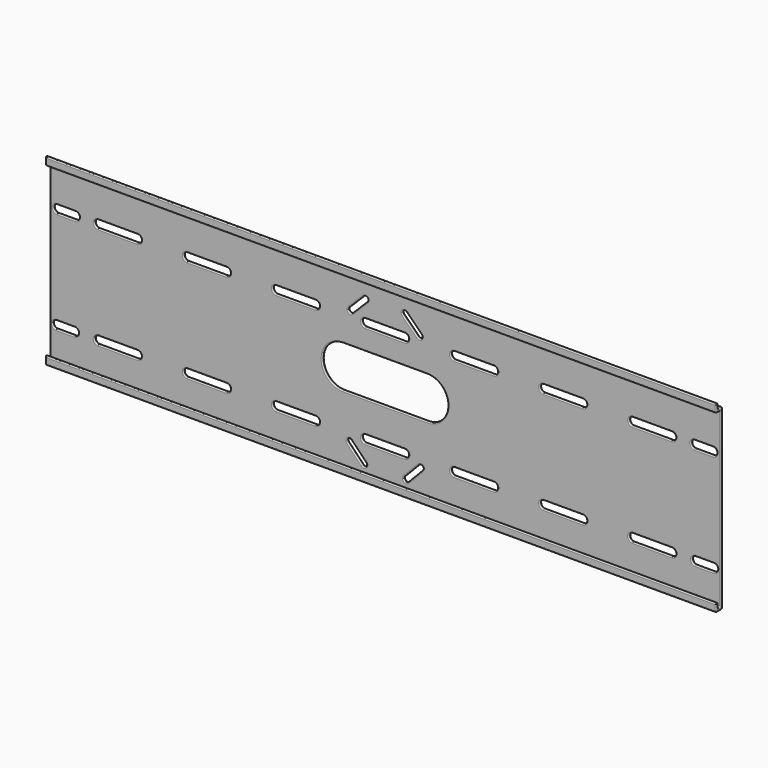
from build123d import *

# Parameters (mm, degrees)
F0_W     = 812.8
F0_H     = 222.25
F1_DEPTH = 9.525
F2_W     = 3.175
F2_H     = 6.35
F2_W_2   = 6.35
F3_DEPTH = 812.801
F5_DEPTH = 9.526
F6_F1_R  = 1.27
F6_F2_R  = 1.27


with BuildPart() as f1:
    # F0 (on Front) → F1 (new body)
    with BuildSketch(Plane.XZ):
        with Locations((103.5543584931, 7.2905048728)):
            Rectangle(F0_W, F0_H)
        with BuildLine():
            ThreePointArc((-294.9081415069, -65.7344951272), (-299.6706415069, -60.9719951272), (-294.9081415069, -56.2094951272))
            Line((-294.9081415069, -56.2094951272), (-272.6831415069, -56.2094951272))
            ThreePointArc((-272.6831415069, -56.2094951272), (-269.3155454615, -57.6043990818), (-267.9206415069, -60.9719951272))
            ThreePointArc((-267.9206415069, -60.9719951272), (-269.3155454615, -64.3395911726), (-272.6831415069, -65.7344951272))
            Line((-272.6831415069, -65.7344951272), (-294.9081415069, -65.7344951272))
        make_face(mode=Mode.SUBTRACT)
        with BuildLine():
            ThreePointArc((-191.7550515069, -60.9719951272), (-193.1499554615, -64.3395911726), (-196.5175515069, -65.7344951272))
            Line((-196.5175515069, -65.7344951272), (-244.1425515069, -65.7344951272))
            ThreePointArc((-244.1425515069, -65.7344951272), (-248.9050515069, -60.9719951272), (-244.1425515069, -56.2094951272))
            Line((-244.1425515069, -56.2094951272), (-196.5175515069, -56.2094951272))
            ThreePointArc((-196.5175515069, -56.2094951272), (-193.1499554615, -57.6043990818), (-191.7550515069, -60.9719951272))
        make_face(mode=Mode.SUBTRACT)
        with BuildLine():
            ThreePointArc((-83.7935815069, -60.9719951272), (-85.1884854615, -64.3395911726), (-88.5560815069, -65.7344951272))
            Line((-88.5560815069, -65.7344951272), (-136.1810815069, -65.7344951272))
            ThreePointArc((-136.1810815069, -65.7344951272), (-140.9435815069, -60.9719951272), (-136.1810815069, -56.2094951272))
            Line((-136.1810815069, -56.2094951272), (-88.5560815069, -56.2094951272))
            ThreePointArc((-88.5560815069, -56.2094951272), (-85.1884854615, -57.6043990818), (-83.7935815069, -60.9719951272))
        make_face(mode=Mode.SUBTRACT)
        with BuildLine():
            ThreePointArc((24.1678884931, -60.9719951272), (22.7729845385, -64.3395911726), (19.4053884931, -65.7344951272))
            Line((19.4053884931, -65.7344951272), (-28.2196115069, -65.7344951272))
            ThreePointArc((-28.2196115069, -65.7344951272), (-32.9821115069, -60.9719951272), (-28.2196115069, -56.2094951272))
            Line((-28.2196115069, -56.2094951272), (19.4053884931, -56.2094951272))
            ThreePointArc((19.4053884931, -56.2094951272), (22.7729845385, -57.6043990818), (24.1678884931, -60.9719951272))
        make_face(mode=Mode.SUBTRACT)
        with BuildLine():
            ThreePointArc((79.7418584931, -65.7344951272), (74.9793584931, -60.9719951272), (79.7418584931, -56.2094951272))
            Line((79.7418584931, -56.2094951272), (127.3668584931, -56.2094951272))
            ThreePointArc((127.3668584931, -56.2094951272), (130.7344545385, -57.6043990818), (132.1293584931, -60.9719951272))
            ThreePointArc((132.1293584931, -60.9719951272), (130.7344545385, -64.3395911726), (127.3668584931, -65.7344951272))
            Line((127.3668584931, -65.7344951272), (79.7418584931, -65.7344951272))
        make_face(mode=Mode.SUBTRACT)
        with BuildLine():
            Line((187.7033284931, -56.2094951272), (235.3283284931, -56.2094951272))
            ThreePointArc((235.3283284931, -56.2094951272), (238.6959245385, -57.6043990818), (240.0908284931, -60.9719951272))
            ThreePointArc((240.0908284931, -60.9719951272), (238.6959245385, -64.3395911726), (235.3283284931, -65.7344951272))
            Line((235.3283284931, -65.7344951272), (187.7033284931, -65.7344951272))
            ThreePointArc((187.7033284931, -65.7344951272), (182.9408284931, -60.9719951272), (187.7033284931, -56.2094951272))
        make_face(mode=Mode.SUBTRACT)
        with BuildLine():
            ThreePointArc((343.2897984931, -56.2094951272), (346.6573945385, -57.6043990818), (348.0522984931, -60.9719951272))
            ThreePointArc((348.0522984931, -60.9719951272), (346.6573945385, -64.3395911726), (343.2897984931, -65.7344951272))
            Line((343.2897984931, -65.7344951272), (295.6647984931, -65.7344951272))
            ThreePointArc((295.6647984931, -65.7344951272), (290.9022984931, -60.9719951272), (295.6647984931, -56.2094951272))
            Line((295.6647984931, -56.2094951272), (343.2897984931, -56.2094951272))
        make_face(mode=Mode.SUBTRACT)
        with BuildLine():
            ThreePointArc((451.2512684931, -56.2094951272), (454.6188645385, -57.6043990818), (456.0137684931, -60.9719951272))
            ThreePointArc((456.0137684931, -60.9719951272), (454.6188645385, -64.3395911726), (451.2512684931, -65.7344951272))
            Line((451.2512684931, -65.7344951272), (403.6262684931, -65.7344951272))
            ThreePointArc((403.6262684931, -65.7344951272), (398.8637684931, -60.9719951272), (403.6262684931, -56.2094951272))
            Line((403.6262684931, -56.2094951272), (451.2512684931, -56.2094951272))
        make_face(mode=Mode.SUBTRACT)
        with BuildLine():
            Line((479.7918584931, -56.2094951272), (502.0168584931, -56.2094951272))
            ThreePointArc((502.0168584931, -56.2094951272), (505.3844545385, -57.6043990818), (506.7793584931, -60.9719951272))
            ThreePointArc((506.7793584931, -60.9719951272), (505.3844545385, -64.3395911726), (502.0168584931, -65.7344951272))
            Line((502.0168584931, -65.7344951272), (479.7918584931, -65.7344951272))
            ThreePointArc((479.7918584931, -65.7344951272), (475.0293584931, -60.9719951272), (479.7918584931, -56.2094951272))
        make_face(mode=Mode.SUBTRACT)
        with BuildLine():
            ThreePointArc((-293.891865778, 58.0905048728), (-298.654365778, 62.8530048728), (-293.891865778, 67.6155048728))
            Line((-293.891865778, 67.6155048728), (-271.666865778, 67.6155048728))
            ThreePointArc((-271.666865778, 67.6155048728), (-268.2992697326, 66.2206009182), (-266.904365778, 62.8530048728))
            ThreePointArc((-266.904365778, 62.8530048728), (-268.2992697326, 59.4854088274), (-271.666865778, 58.0905048728))
            Line((-271.666865778, 58.0905048728), (-293.891865778, 58.0905048728))
        make_face(mode=Mode.SUBTRACT)
        with BuildLine():
            ThreePointArc((-196.4831415069, 67.6155048728), (-193.1155454615, 66.2206009182), (-191.7206415069, 62.8530048728))
            ThreePointArc((-191.7206415069, 62.8530048728), (-193.1155454615, 59.4854088274), (-196.4831415069, 58.0905048728))
            Line((-196.4831415069, 58.0905048728), (-244.1081415069, 58.0905048728))
            ThreePointArc((-244.1081415069, 58.0905048728), (-248.8706415069, 62.8530048728), (-244.1081415069, 67.6155048728))
            Line((-244.1081415069, 67.6155048728), (-196.4831415069, 67.6155048728))
        make_face(mode=Mode.SUBTRACT)
        with BuildLine():
            ThreePointArc((-88.5331415069, 67.6155048728), (-85.1655454615, 66.2206009182), (-83.7706415069, 62.8530048728))
            ThreePointArc((-83.7706415069, 62.8530048728), (-85.1655454615, 59.4854088274), (-88.5331415069, 58.0905048728))
            Line((-88.5331415069, 58.0905048728), (-136.1581415069, 58.0905048728))
            ThreePointArc((-136.1581415069, 58.0905048728), (-140.9206415069, 62.8530048728), (-136.1581415069, 67.6155048728))
            Line((-136.1581415069, 67.6155048728), (-88.5331415069, 67.6155048728))
        make_face(mode=Mode.SUBTRACT)
        with BuildLine():
            ThreePointArc((19.4168584931, 67.6155048728), (22.7844545385, 66.2206009182), (24.1793584931, 62.8530048728))
            ThreePointArc((24.1793584931, 62.8530048728), (22.7844545385, 59.4854088274), (19.4168584931, 58.0905048728))
            Line((19.4168584931, 58.0905048728), (-28.2081415069, 58.0905048728))
            ThreePointArc((-28.2081415069, 58.0905048728), (-32.9706415069, 62.8530048728), (-28.2081415069, 67.6155048728))
            Line((-28.2081415069, 67.6155048728), (19.4168584931, 67.6155048728))
        make_face(mode=Mode.SUBTRACT)
        with BuildLine():
            ThreePointArc((52.7543584931, -18.1094951272), (27.3543584931, 7.2905048728), (52.7543584931, 32.6905048728))
            Line((52.7543584931, 32.6905048728), (154.3543584931, 32.6905048728))
            ThreePointArc((154.3543584931, 32.6905048728), (172.3148707352, 25.2510171149), (179.7543584931, 7.2905048728))
            ThreePointArc((179.7543584931, 7.2905048728), (172.3148707352, -10.6700073693), (154.3543584931, -18.1094951272))
            Line((154.3543584931, -18.1094951272), (52.7543584931, -18.1094951272))
        make_face(mode=Mode.SUBTRACT)
        with BuildLine():
            ThreePointArc((79.7418584931, 58.0905048728), (74.9793584931, 62.8530048728), (79.7418584931, 67.6155048728))
            Line((79.7418584931, 67.6155048728), (127.3668584931, 67.6155048728))
            ThreePointArc((127.3668584931, 67.6155048728), (130.7344545385, 66.2206009182), (132.1293584931, 62.8530048728))
            ThreePointArc((132.1293584931, 62.8530048728), (130.7344545385, 59.4854088274), (127.3668584931, 58.0905048728))
            Line((127.3668584931, 58.0905048728), (79.7418584931, 58.0905048728))
        make_face(mode=Mode.SUBTRACT)
        with BuildLine():
            ThreePointArc((187.6918584931, 58.0905048728), (182.9293584931, 62.8530048728), (187.6918584931, 67.6155048728))
            Line((187.6918584931, 67.6155048728), (235.3168584931, 67.6155048728))
            ThreePointArc((235.3168584931, 67.6155048728), (238.6844545385, 66.2206009182), (240.0793584931, 62.8530048728))
            ThreePointArc((240.0793584931, 62.8530048728), (238.6844545385, 59.4854088274), (235.3168584931, 58.0905048728))
            Line((235.3168584931, 58.0905048728), (187.6918584931, 58.0905048728))
        make_face(mode=Mode.SUBTRACT)
        with BuildLine():
            ThreePointArc((295.6418584931, 58.0905048728), (290.8793584931, 62.8530048728), (295.6418584931, 67.6155048728))
            Line((295.6418584931, 67.6155048728), (343.2668584931, 67.6155048728))
            ThreePointArc((343.2668584931, 67.6155048728), (346.6344545385, 66.2206009182), (348.0293584931, 62.8530048728))
            ThreePointArc((348.0293584931, 62.8530048728), (346.6344545385, 59.4854088274), (343.2668584931, 58.0905048728))
            Line((343.2668584931, 58.0905048728), (295.6418584931, 58.0905048728))
        make_face(mode=Mode.SUBTRACT)
        with BuildLine():
            ThreePointArc((451.2168584931, 67.6155048728), (454.5844545385, 66.2206009182), (455.9793584931, 62.8530048728))
            ThreePointArc((455.9793584931, 62.8530048728), (454.5844545385, 59.4854088274), (451.2168584931, 58.0905048728))
            Line((451.2168584931, 58.0905048728), (403.5918584931, 58.0905048728))
            ThreePointArc((403.5918584931, 58.0905048728), (398.8293584931, 62.8530048728), (403.5918584931, 67.6155048728))
            Line((403.5918584931, 67.6155048728), (451.2168584931, 67.6155048728))
        make_face(mode=Mode.SUBTRACT)
        with BuildLine():
            ThreePointArc((478.7755827641, 58.0905048728), (474.0130827641, 62.8530048728), (478.7755827641, 67.6155048728))
            Line((478.7755827641, 67.6155048728), (501.0005827641, 67.6155048728))
            ThreePointArc((501.0005827641, 67.6155048728), (504.3681788095, 66.2206009182), (505.7630827641, 62.8530048728))
            ThreePointArc((505.7630827641, 62.8530048728), (504.3681788095, 59.4854088274), (501.0005827641, 58.0905048728))
            Line((501.0005827641, 58.0905048728), (478.7755827641, 58.0905048728))
        make_face(mode=Mode.SUBTRACT)
    extrude(amount=F1_DEPTH)

    # F2 (on face) → F3 (cut, through all)
    with BuildSketch(Plane(origin=(-302.8456415069, 0, 0), x_dir=(0, -1, 0), z_dir=(-1, 0, 0))):
        with Locations((4.7625, -97.4844951272)):
            Rectangle(F2_W, F2_H)
        Polygon((9.525, -94.3094951272), (9.525, 108.8905048728), (3.175, 108.8905048728), (3.175, -94.3094951272), (6.35, -94.3094951272), align=None)
        with Locations((3.175, 115.2405048728)):
            Rectangle(F2_W_2, F2_H)
    extrude(amount=-F3_DEPTH, mode=Mode.SUBTRACT)

    # F4 (on face) → F5 (cut, through all)
    with BuildSketch(Plane(origin=(0, 0, 0), x_dir=(-1, 0, 0), z_dir=(0, 1, 0))):
        with BuildLine():
            ThreePointArc((-125.1217944628, 86.0079408425), (-124.4335409773, 87.037984975), (-124.1918584931, 88.2530048728))
            ThreePointArc((-124.1918584931, 88.2530048728), (-126.1518385953, 91.1863223885), (-129.6119225233, 90.4980689031))
            ThreePointArc((-129.6119225233, 90.4980689031), (-129.6119225233, 86.0079408425), (-125.1217944628, 86.0079408425))
        make_face()
        with BuildLine():
            ThreePointArc((-125.1217944628, 86.0079408425), (-129.6119225233, 86.0079408425), (-129.6119225233, 90.4980689031))
            Line((-129.6119225233, 90.4980689031), (-147.5724347655, 72.5375566609))
            ThreePointArc((-147.5724347655, 72.5375566609), (-144.1123508374, 73.2258101464), (-142.1523707352, 70.2924926307))
            ThreePointArc((-142.1523707352, 70.2924926307), (-142.3940532195, 69.0774727329), (-143.0823067049, 68.0474286004))
            Line((-143.0823067049, 68.0474286004), (-125.1217944628, 86.0079408425))
        make_face()
        with BuildLine():
            ThreePointArc((-142.1523707352, 70.2924926307), (-144.1123508374, 73.2258101464), (-147.5724347655, 72.5375566609))
            ThreePointArc((-147.5724347655, 72.5375566609), (-147.5724347655, 68.0474286004), (-143.0823067049, 68.0474286004))
            ThreePointArc((-143.0823067049, 68.0474286004), (-142.3940532195, 69.0774727329), (-142.1523707352, 70.2924926307))
        make_face()
        with BuildLine():
            ThreePointArc((-81.9869225233, 86.0079408425), (-78.5268385953, 85.3196873571), (-76.5668584931, 88.2530048728))
            ThreePointArc((-76.5668584931, 88.2530048728), (-76.8085409773, 89.4680247706), (-77.4967944628, 90.4980689031))
            ThreePointArc((-77.4967944628, 90.4980689031), (-81.9869225233, 90.4980689031), (-81.9869225233, 86.0079408425))
        make_face()
        with BuildLine():
            ThreePointArc((-77.4967944628, 90.4980689031), (-76.8085409773, 89.4680247706), (-76.5668584931, 88.2530048728))
            ThreePointArc((-76.5668584931, 88.2530048728), (-78.5268385953, 85.3196873571), (-81.9869225233, 86.0079408425))
            Line((-81.9869225233, 86.0079408425), (-64.0264102812, 68.0474286004))
            ThreePointArc((-64.0264102812, 68.0474286004), (-64.0264102812, 72.5375566609), (-59.5362822207, 72.5375566609))
            Line((-59.5362822207, 72.5375566609), (-77.4967944628, 90.4980689031))
        make_face()
        with BuildLine():
            ThreePointArc((-58.6063462509, 70.2924926307), (-58.8480287352, 71.5075125284), (-59.5362822207, 72.5375566609))
            ThreePointArc((-59.5362822207, 72.5375566609), (-64.0264102812, 72.5375566609), (-64.0264102812, 68.0474286004))
            ThreePointArc((-64.0264102812, 68.0474286004), (-60.5663263532, 67.3591751149), (-58.6063462509, 70.2924926307))
        make_face()
        with BuildLine():
            ThreePointArc((-143.4957509266, -69.9355006927), (-143.7259286835, -68.7486363549), (-144.383087592, -67.7338600618))
            ThreePointArc((-144.383087592, -67.7338600618), (-148.8723915575, -67.6478373582), (-148.9584142612, -72.1371413237))
            ThreePointArc((-148.9584142612, -72.1371413237), (-145.4838865888, -72.8803229359), (-143.4957509266, -69.9355006927))
        make_face()
        with BuildLine():
            ThreePointArc((-131.3452892139, -90.4384480002), (-131.2592665102, -85.9491440347), (-126.7699625448, -86.0351667384))
            Line((-126.7699625448, -86.0351667384), (-144.383087592, -67.7338600618))
            ThreePointArc((-144.383087592, -67.7338600618), (-143.7259286835, -68.7486363549), (-143.4957509266, -69.9355006927))
            ThreePointArc((-143.4957509266, -69.9355006927), (-145.4838865888, -72.8803229359), (-148.9584142612, -72.1371413237))
            Line((-148.9584142612, -72.1371413237), (-131.3452892139, -90.4384480002))
        make_face()
        with BuildLine():
            ThreePointArc((-125.8826258793, -88.2368073693), (-126.1128036362, -87.0499430315), (-126.7699625448, -86.0351667384))
            ThreePointArc((-126.7699625448, -86.0351667384), (-131.2592665102, -85.9491440347), (-131.3452892139, -90.4384480002))
            ThreePointArc((-131.3452892139, -90.4384480002), (-127.8707615415, -91.1816296124), (-125.8826258793, -88.2368073693))
        make_face()
        with BuildLine():
            ThreePointArc((-80.3387544414, -86.0351667384), (-80.2527317377, -90.5244707038), (-75.7634277722, -90.4384480002))
            ThreePointArc((-75.7634277722, -90.4384480002), (-75.1062688637, -89.4236717071), (-74.8760911068, -88.2368073693))
            ThreePointArc((-74.8760911068, -88.2368073693), (-76.864226769, -85.2919851262), (-80.3387544414, -86.0351667384))
        make_face()
        with BuildLine():
            ThreePointArc((-74.8760911068, -88.2368073693), (-75.1062688637, -89.4236717071), (-75.7634277722, -90.4384480002))
            Line((-75.7634277722, -90.4384480002), (-58.1503027249, -72.1371413237))
            ThreePointArc((-58.1503027249, -72.1371413237), (-62.6396066904, -72.2231640273), (-62.7256293941, -67.7338600618))
            Line((-62.7256293941, -67.7338600618), (-80.3387544414, -86.0351667384))
            ThreePointArc((-80.3387544414, -86.0351667384), (-76.864226769, -85.2919851262), (-74.8760911068, -88.2368073693))
        make_face()
        with BuildLine():
            ThreePointArc((-62.7256293941, -67.7338600618), (-62.6396066904, -72.2231640273), (-58.1503027249, -72.1371413237))
            ThreePointArc((-58.1503027249, -72.1371413237), (-57.4931438164, -71.1223650306), (-57.2629660595, -69.9355006927))
            ThreePointArc((-57.2629660595, -69.9355006927), (-59.2511017217, -66.9906784496), (-62.7256293941, -67.7338600618))
        make_face()
    extrude(amount=-F5_DEPTH, mode=Mode.SUBTRACT)

    # F6: fillet of radius 1.27 on 212 edges, made by hand

    # F6_f1
    f6_f1_edges = [f1.edges().sort_by_distance(p)[0] for p in [
        (103.5543584931, -3.175, 108.8905048728),
        (103.5543584931, -3.175, -100.6594951272),
        (103.5543584931, -6.35, 112.0655048728),
        (103.5543584931, -6.35, -100.6594951272),
    ]]
    fillet(f6_f1_edges, radius=F6_F1_R)

    # F6_f2
    f6_f2_edges = [f1.edges().sort_by_distance(p)[0] for p in [
        (-302.8456415069, -3.175, 4.1155048728),
        (509.9543584931, -3.175, 4.1155048728),
        (474.0130827641, -3.175, 62.8530048728),
        (489.8880827641, -3.175, 58.0905048728),
        (489.8880827641, -3.175, 67.6155048728),
        (505.7630827641, -3.175, 62.8530048728),
        (398.8293584931, -3.175, 62.8530048728),
        (427.4043584931, -3.175, 58.0905048728),
        (427.4043584931, -3.175, 67.6155048728),
        (455.9793584931, -3.175, 62.8530048728),
        (348.0293584931, -3.175, 62.8530048728),
        (319.4543584931, -3.175, 67.6155048728),
        (319.4543584931, -3.175, 58.0905048728),
        (290.8793584931, -3.175, 62.8530048728),
        (182.9293584931, -3.175, 62.8530048728),
        (211.5043584931, -3.175, 58.0905048728),
        (211.5043584931, -3.175, 67.6155048728),
        (240.0793584931, -3.175, 62.8530048728),
        (125.1217944628, -3.175, 90.4980689031),
        (138.5921786444, -3.175, 81.517812782),
        (147.5724347655, -3.175, 68.0474286004),
        (134.1020505839, -3.175, 77.0276847215),
        (74.9793584931, -3.175, 62.8530048728),
        (103.5543584931, -3.175, 58.0905048728),
        (103.5543584931, -3.175, 67.6155048728),
        (132.1293584931, -3.175, 62.8530048728),
        (475.0293584931, -3.175, -60.9719951272),
        (490.9043584931, -3.175, -65.7344951272),
        (490.9043584931, -3.175, -56.2094951272),
        (506.7793584931, -3.175, -60.9719951272),
        (456.0137684931, -3.175, -60.9719951272),
        (427.4387684931, -3.175, -56.2094951272),
        (427.4387684931, -3.175, -65.7344951272),
        (398.8637684931, -3.175, -60.9719951272),
        (290.9022984931, -3.175, -60.9719951272),
        (319.4772984931, -3.175, -65.7344951272),
        (319.4772984931, -3.175, -56.2094951272),
        (348.0522984931, -3.175, -60.9719951272),
        (182.9408284931, -3.175, -60.9719951272),
        (211.5158284931, -3.175, -65.7344951272),
        (211.5158284931, -3.175, -56.2094951272),
        (240.0908284931, -3.175, -60.9719951272),
        (148.8723915575, -3.175, -67.6478373582),
        (140.1518517375, -3.175, -81.2877946619),
        (126.8559852484, -3.175, -90.5244707038),
        (135.5765250684, -3.175, -76.8845134001),
        (81.9869225233, -3.175, 90.4980689031),
        (73.0066664023, -3.175, 77.0276847215),
        (59.5362822207, -3.175, 68.0474286004),
        (68.5165383417, -3.175, 81.517812782),
        (24.1793584931, -3.175, 62.8530048728),
        (-4.3956415069, -3.175, 67.6155048728),
        (-4.3956415069, -3.175, 58.0905048728),
        (-32.9706415069, -3.175, 62.8530048728),
        (27.3543584931, -3.175, 7.2905048728),
        (103.5543584931, -3.175, -18.1094951272),
        (103.5543584931, -3.175, 32.6905048728),
        (179.7543584931, -3.175, 7.2905048728),
        (-140.9206415069, -3.175, 62.8530048728),
        (-112.3456415069, -3.175, 58.0905048728),
        (-112.3456415069, -3.175, 67.6155048728),
        (-83.7706415069, -3.175, 62.8530048728),
        (-248.8706415069, -3.175, 62.8530048728),
        (-220.2956415069, -3.175, 58.0905048728),
        (-220.2956415069, -3.175, 67.6155048728),
        (-191.7206415069, -3.175, 62.8530048728),
        (-266.904365778, -3.175, 62.8530048728),
        (-282.779365778, -3.175, 67.6155048728),
        (-282.779365778, -3.175, 58.0905048728),
        (-298.654365778, -3.175, 62.8530048728),
        (132.1293584931, -3.175, -60.9719951272),
        (103.5543584931, -3.175, -56.2094951272),
        (103.5543584931, -3.175, -65.7344951272),
        (74.9793584931, -3.175, -60.9719951272),
        (80.2527317377, -3.175, -90.5244707038),
        (66.9568652486, -3.175, -81.2877946619),
        (58.2363254286, -3.175, -67.6478373582),
        (71.5321919177, -3.175, -76.8845134001),
        (24.1678884931, -3.175, -60.9719951272),
        (-4.4071115069, -3.175, -56.2094951272),
        (-4.4071115069, -3.175, -65.7344951272),
        (-32.9821115069, -3.175, -60.9719951272),
        (-83.7935815069, -3.175, -60.9719951272),
        (-112.3685815069, -3.175, -56.2094951272),
        (-112.3685815069, -3.175, -65.7344951272),
        (-140.9435815069, -3.175, -60.9719951272),
        (-191.7550515069, -3.175, -60.9719951272),
        (-220.3300515069, -3.175, -56.2094951272),
        (-220.3300515069, -3.175, -65.7344951272),
        (-248.9050515069, -3.175, -60.9719951272),
        (-299.6706415069, -3.175, -60.9719951272),
        (-283.7956415069, -3.175, -65.7344951272),
        (-283.7956415069, -3.175, -56.2094951272),
        (-267.9206415069, -3.175, -60.9719951272),
        (509.9543584931, 0, 4.1155048728),
        (103.5543584931, 0, -103.8344951272),
        (103.5543584931, 0, 112.0655048728),
        (-302.8456415069, 0, 4.1155048728),
        (-299.6706415069, 0, -60.9719951272),
        (-283.7956415069, 0, -65.7344951272),
        (-283.7956415069, 0, -56.2094951272),
        (-267.9206415069, 0, -60.9719951272),
        (-191.7550515069, 0, -60.9719951272),
        (-220.3300515069, 0, -56.2094951272),
        (-220.3300515069, 0, -65.7344951272),
        (-248.9050515069, 0, -60.9719951272),
        (-83.7935815069, 0, -60.9719951272),
        (-112.3685815069, 0, -56.2094951272),
        (-112.3685815069, 0, -65.7344951272),
        (-140.9435815069, 0, -60.9719951272),
        (71.5321919177, 0, -76.8845134001),
        (58.2363254286, 0, -67.6478373582),
        (66.9568652486, 0, -81.2877946619),
        (80.2527317377, 0, -90.5244707038),
        (24.1678884931, 0, -60.9719951272),
        (-4.4071115069, 0, -56.2094951272),
        (-4.4071115069, 0, -65.7344951272),
        (-32.9821115069, 0, -60.9719951272),
        (135.5765250684, 0, -76.8845134001),
        (126.8559852484, 0, -90.5244707038),
        (140.1518517375, 0, -81.2877946619),
        (148.8723915575, 0, -67.6478373582),
        (103.5543584931, 0, -65.7344951272),
        (132.1293584931, 0, -60.9719951272),
        (74.9793584931, 0, -60.9719951272),
        (103.5543584931, 0, -56.2094951272),
        (211.5158284931, 0, -56.2094951272),
        (182.9408284931, 0, -60.9719951272),
        (240.0908284931, 0, -60.9719951272),
        (211.5158284931, 0, -65.7344951272),
        (290.9022984931, 0, -60.9719951272),
        (319.4772984931, 0, -65.7344951272),
        (319.4772984931, 0, -56.2094951272),
        (348.0522984931, 0, -60.9719951272),
        (456.0137684931, 0, -60.9719951272),
        (427.4387684931, 0, -56.2094951272),
        (427.4387684931, 0, -65.7344951272),
        (398.8637684931, 0, -60.9719951272),
        (475.0293584931, 0, -60.9719951272),
        (490.9043584931, 0, -65.7344951272),
        (490.9043584931, 0, -56.2094951272),
        (506.7793584931, 0, -60.9719951272),
        (-282.779365778, 0, 58.0905048728),
        (-266.904365778, 0, 62.8530048728),
        (-298.654365778, 0, 62.8530048728),
        (-282.779365778, 0, 67.6155048728),
        (-248.8706415069, 0, 62.8530048728),
        (-220.2956415069, 0, 58.0905048728),
        (-220.2956415069, 0, 67.6155048728),
        (-191.7206415069, 0, 62.8530048728),
        (-140.9206415069, 0, 62.8530048728),
        (-112.3456415069, 0, 58.0905048728),
        (-112.3456415069, 0, 67.6155048728),
        (-83.7706415069, 0, 62.8530048728),
        (-4.3956415069, 0, 58.0905048728),
        (24.1793584931, 0, 62.8530048728),
        (-32.9706415069, 0, 62.8530048728),
        (-4.3956415069, 0, 67.6155048728),
        (68.5165383417, 0, 81.517812782),
        (59.5362822207, 0, 68.0474286004),
        (73.0066664023, 0, 77.0276847215),
        (81.9869225233, 0, 90.4980689031),
        (27.3543584931, 0, 7.2905048728),
        (103.5543584931, 0, -18.1094951272),
        (103.5543584931, 0, 32.6905048728),
        (179.7543584931, 0, 7.2905048728),
        (74.9793584931, 0, 62.8530048728),
        (103.5543584931, 0, 58.0905048728),
        (103.5543584931, 0, 67.6155048728),
        (132.1293584931, 0, 62.8530048728),
        (182.9293584931, 0, 62.8530048728),
        (211.5043584931, 0, 58.0905048728),
        (211.5043584931, 0, 67.6155048728),
        (240.0793584931, 0, 62.8530048728),
        (134.1020505839, 0, 77.0276847215),
        (147.5724347655, 0, 68.0474286004),
        (138.5921786444, 0, 81.517812782),
        (125.1217944628, 0, 90.4980689031),
        (319.4543584931, 0, 58.0905048728),
        (348.0293584931, 0, 62.8530048728),
        (290.8793584931, 0, 62.8530048728),
        (319.4543584931, 0, 67.6155048728),
        (398.8293584931, 0, 62.8530048728),
        (427.4043584931, 0, 58.0905048728),
        (427.4043584931, 0, 67.6155048728),
        (455.9793584931, 0, 62.8530048728),
        (474.0130827641, 0, 62.8530048728),
        (489.8880827641, 0, 58.0905048728),
        (489.8880827641, 0, 67.6155048728),
        (505.7630827641, 0, 62.8530048728),
        (509.9543584931, -9.525, 113.6530048728),
        (103.5543584931, -9.525, 108.8905048728),
        (-302.8456415069, -9.525, 113.6530048728),
        (103.5543584931, -9.525, 118.4155048728),
        (-302.8456415069, -2.54, 112.0655048728),
        (509.9543584931, -2.54, 112.0655048728),
        (-302.8456415069, -6.35, 115.8755048728),
        (103.5543584931, -6.35, 118.4155048728),
        (509.9543584931, -6.35, 115.8755048728),
        (-302.8456415069, -6.35, -96.8494951272),
        (103.5543584931, -6.35, -94.3094951272),
        (509.9543584931, -6.35, -96.8494951272),
        (509.9543584931, -9.525, -99.0719951272),
        (103.5543584931, -9.525, -103.8344951272),
        (-302.8456415069, -9.525, -99.0719951272),
        (103.5543584931, -9.525, -94.3094951272),
        (-302.8456415069, -4.7625, -103.8344951272),
        (509.9543584931, -4.7625, -103.8344951272),
        (509.9543584931, -5.9780256121, -100.2875207393),
        (-302.8456415069, -5.9780256121, -100.2875207393),
        (509.9543584931, -5.9780256121, 112.4374792607),
        (-302.8456415069, -5.9780256121, 112.4374792607),
        (509.9543584931, -3.5469743879, 108.5185304849),
        (509.9543584931, -3.5469743879, -100.2875207393),
        (-302.8456415069, -3.5469743879, 108.5185304849),
        (-302.8456415069, -3.5469743879, -100.2875207393),
    ]]
    fillet(f6_f2_edges, radius=F6_F2_R)


solid = f1.part
